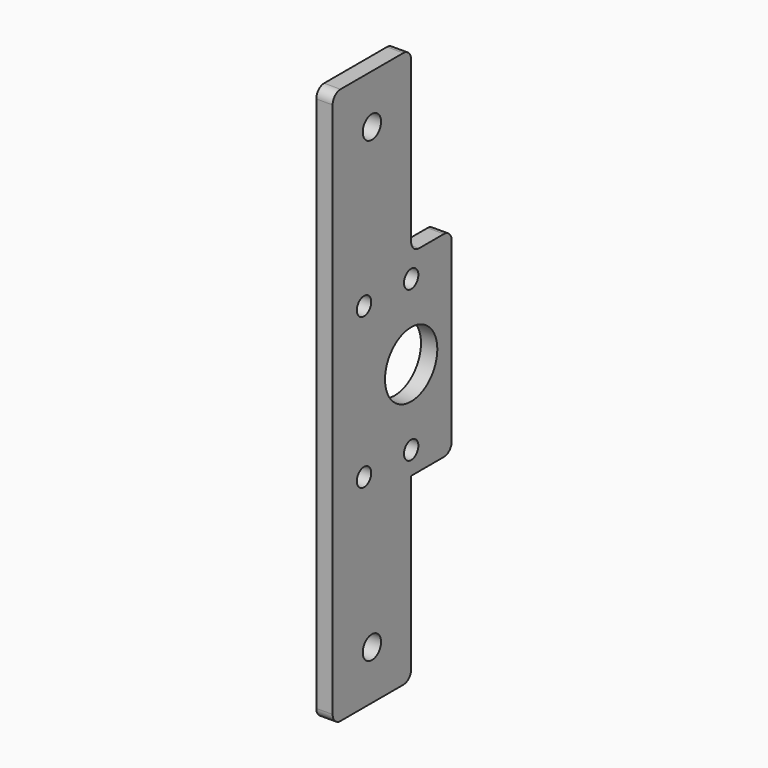
from build123d import *

# Parameters (mm, degrees)
F1_DEPTH = 5
F2_R     = 3
F3_R     = 3.5
F4_DEPTH = 5
F6_R     = 10
F6_R_2   = 2.75
F7_DEPTH = 5


# Not quite as in the source:
# - two fillets or chamfers of one size are made in one step


with BuildPart() as f1:
    # F0 (on Right) → F1 (new body)
    with BuildSketch(Plane.YZ):
        Polygon((15, 30), (15, 85), (-15, 85), (-15, -85), (15, -85), (15, -30), (30.5, -30), (30.5, 30), align=None)
    extrude(amount=F1_DEPTH)

    # F2
    f2_edges = [f1.edges().sort_by_distance(p)[0] for p in [
        (2.5, -15, 85),
        (2.5, 15, 85),
        (2.5, -15, -85),
        (2.5, 15, 30),
        (2.5, 15, -85),
        (2.5, 30.5, -30),
        (2.5, 30.5, 30),
    ]]
    fillet(f2_edges, radius=F2_R)

    # F3 (on face) → F4 (cut)
    with BuildSketch(Plane.YZ.offset(5)):
        with Locations((0, 70)):
            Circle(F3_R)
        with Locations((0, -70)):
            Circle(F3_R)
    extrude(amount=-F4_DEPTH, mode=Mode.SUBTRACT)

    # F6 (on face) → F7 (cut)
    with BuildSketch(Plane.YZ.offset(5)):
        with Locations((15, 0)):
            Circle(F6_R)
        with Locations((15, 23)):
            Circle(F6_R_2)
        with Locations((15, -23)):
            Circle(F6_R_2)
        with Locations((-3, -23)):
            Circle(F6_R_2)
        with Locations((-3, 23)):
            Circle(F6_R_2)
    extrude(amount=-F7_DEPTH, mode=Mode.SUBTRACT)


solid = f1.part
